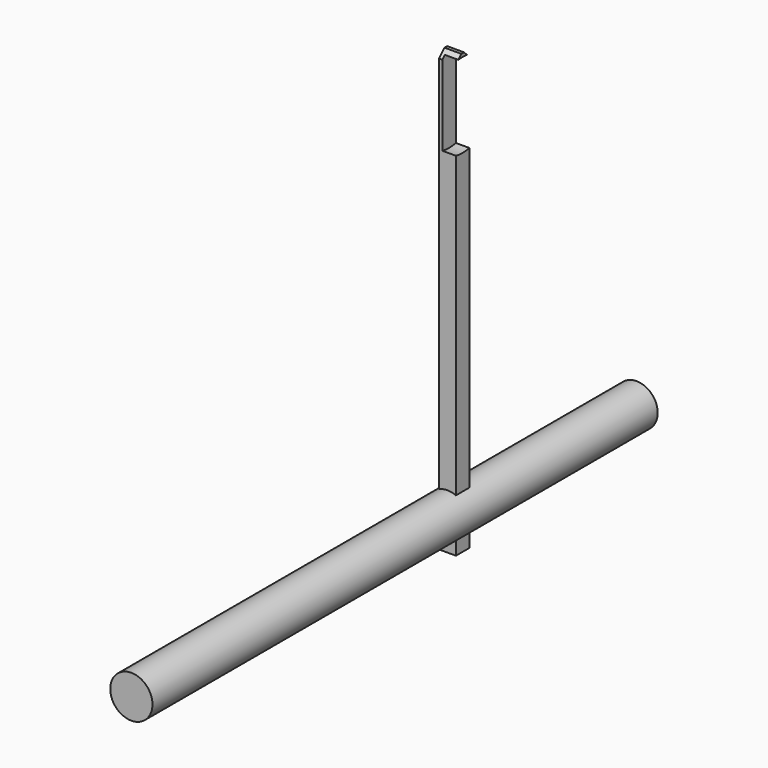
from build123d import *

# Parameters (mm, degrees)
F0_R          = 15.875
F1_DEPTH      = 474.98
F2_W          = 12.7
F2_H          = 12.7
F3_DEPTH      = 15.876
F3_DEPTH_BACK = 15.876
F4_DEPTH      = 304.8
F4_DEPTH_BACK = 25.4
F6_SIZE       = 5.08
F7_DEPTH      = 10.16


with BuildPart() as f1:
    # F0 (on Front) → F1 (new body)
    with BuildSketch(Plane.XZ):
        Circle(F0_R)
    extrude(amount=F1_DEPTH)

    # F2 (on Top) → F3 (cut, two sides)
    with BuildSketch(Plane.XY) as f3_sk:
        with Locations((0, -171.45)):
            Rectangle(F2_W, F2_H)
    extrude(amount=-F3_DEPTH, mode=Mode.SUBTRACT)
    extrude(f3_sk.sketch, amount=F3_DEPTH_BACK, mode=Mode.SUBTRACT)


with BuildPart() as f4:
    # F2 (on Top) → F4 (new body, two sides)
    with BuildSketch(Plane.XY) as f4_sk:
        with Locations((0, -171.45)):
            Rectangle(F2_W, F2_H)
    extrude(amount=F4_DEPTH)
    extrude(f4_sk.sketch, amount=-F4_DEPTH_BACK)

    # F6
    f6_edges = [f4.edges().sort_by_distance(p)[0] for p in [
        (0, -177.8, 304.8),
        (0, -165.1, 304.8),
    ]]
    chamfer(f6_edges, length=F6_SIZE)

    # F5 (on face) → F7 (cut)
    with BuildSketch(Plane.YZ.offset(6.35)):
        with BuildLine():
            Line((-165.1, 239.4014802667), (-165.1, 301.6185197333))
            ThreePointArc((-165.1, 301.6185197333), (-171.45, 302.26), (-177.8, 301.6185197333))
            Line((-177.8, 301.6185197333), (-177.8, 239.4014802667))
            ThreePointArc((-177.8, 239.4014802667), (-171.45, 238.76), (-165.1, 239.4014802667))
        make_face()
    extrude(amount=-F7_DEPTH, mode=Mode.SUBTRACT)


solid = Compound([f1.part, f4.part])
